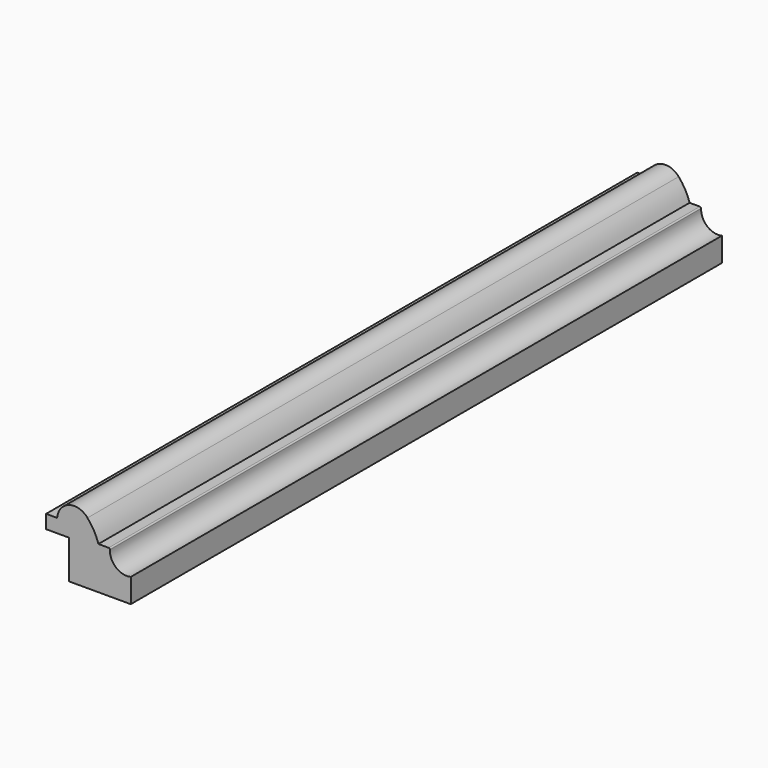
from build123d import *

# Parameters (mm, degrees)
F1_DEPTH = 152.4


# Not quite as in the source:
# - ends of sketch curves that miss each other by under 0.0002 mm in the source are joined


with BuildPart() as f1:
    # F0 (on Front) → F1 (new body)
    with BuildSketch(Plane.XZ):
        with BuildLine():
            Line((-8.73125, 3.7119814), (-8.73125, 0.9179814))
            Line((-8.73125, 0.9179814), (-3.96875, 0.9179814))
            Line((-3.96875, 0.9179814), (-3.96875, -7.0195186))
            Line((-3.96875, -7.0195186), (8.73125, -7.0195186))
            Line((8.73125, -7.0195186), (8.73125, -2.0665186))
            ThreePointArc((8.73125, -2.0665186), (5.7032908876, -1.3612616552), (4.438258034, 1.4787376653))
            ThreePointArc((4.438258034, 1.4787376653), (4.3678620463, 1.6652468114), (4.1844976, 1.7434814))
            Line((4.1844976, 1.7434814), (2.06375, 1.7434814))
            ThreePointArc((2.06375, 1.7434814), (1.1469309524, 3.8652258573), (-0.1916191114, 5.7495426677))
            ThreePointArc((-0.1916191114, 5.7495426677), (-4.0073604602, 6.8451953761), (-6.4452349512, 3.7119803958))
            Line((-6.4452349512, 3.7119803958), (-8.73125, 3.7119814))
        make_face()
    extrude(amount=F1_DEPTH)


solid = f1.part
